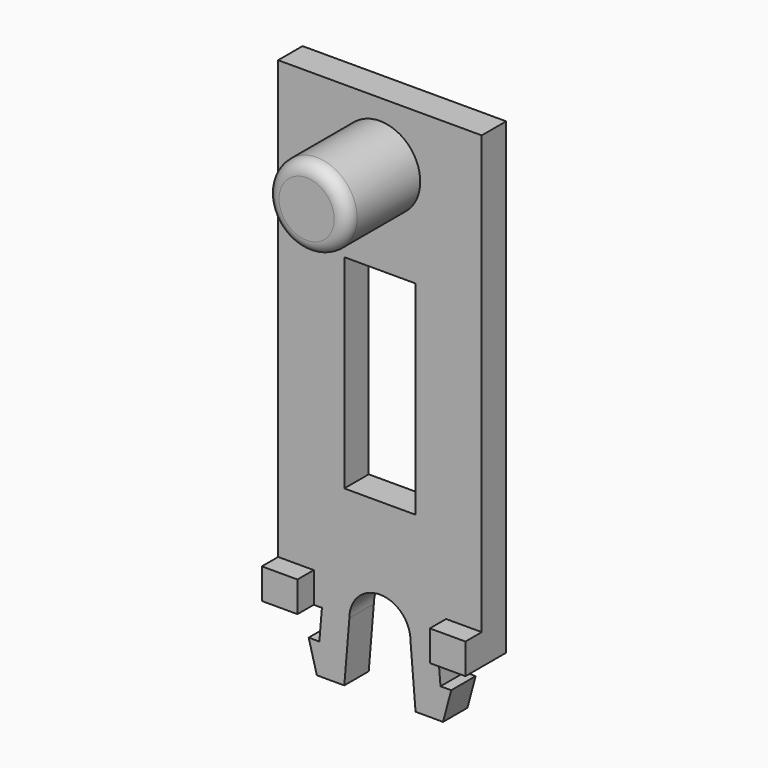
from build123d import *

# Parameters (mm, degrees)
F0_W     = 7
F0_H     = 20
F0_R     = 3.96
F1_DEPTH = 3
F2_R     = 3.96
F3_DEPTH = 12
F4_R     = 1.25
F5_W     = 3.5
F5_H     = 3
F6_DEPTH = 2


with BuildPart() as f1:
    # F0 (on Front) → F1 (new body)
    with BuildSketch(Plane.XZ):
        Polygon((5.7, 0), (3, 0), (3.5, -6), (6.2, -6), (7, -3), (5.95, -3), align=None)
        with BuildLine():
            ThreePointArc((-3, 0), (0, 3), (3, 0))
            Line((3, 0), (5.7, 0))
            Line((5.7, 0), (10, 0))
            Line((10, 0), (10, 45.96))
            Line((10, 45.96), (-10, 45.96))
            Line((-10, 45.96), (-10, 0))
            Line((-10, 0), (-5.7, 0))
            Line((-5.7, 0), (-3, 0))
        make_face()
        with Locations((0, 21.04)):
            Rectangle(F0_W, F0_H, mode=Mode.SUBTRACT)
        with Locations((0, 40)):
            Circle(F0_R, mode=Mode.SUBTRACT)
        Polygon((-3.5, -6), (-3, 0), (-5.7, 0), (-5.95, -3), (-7, -3), (-6.2, -6), align=None)
        with Locations((0, 40)):
            Circle(F0_R)
    extrude(amount=F1_DEPTH)

    # F2 (on face) → F3 (join)
    with BuildSketch(Plane(origin=(0, 0, 0), x_dir=(-1, 0, 0), z_dir=(0, 1, 0))):
        with Locations((0, 40)):
            Circle(F2_R)
    extrude(amount=-F3_DEPTH)

    # F4
    f4_edges = [f1.edges().sort_by_distance(p)[0] for p in [
        (3.96, -12, 40),
    ]]
    fillet(f4_edges, radius=F4_R)

    # F5 (on face) → F6 (join)
    with BuildSketch(Plane.XZ.offset(3)):
        with Locations((-8.25, 1.5)):
            Rectangle(F5_W, F5_H)
        with Locations((8.25, 1.5)):
            Rectangle(F5_W, F5_H)
    extrude(amount=F6_DEPTH)


solid = f1.part
